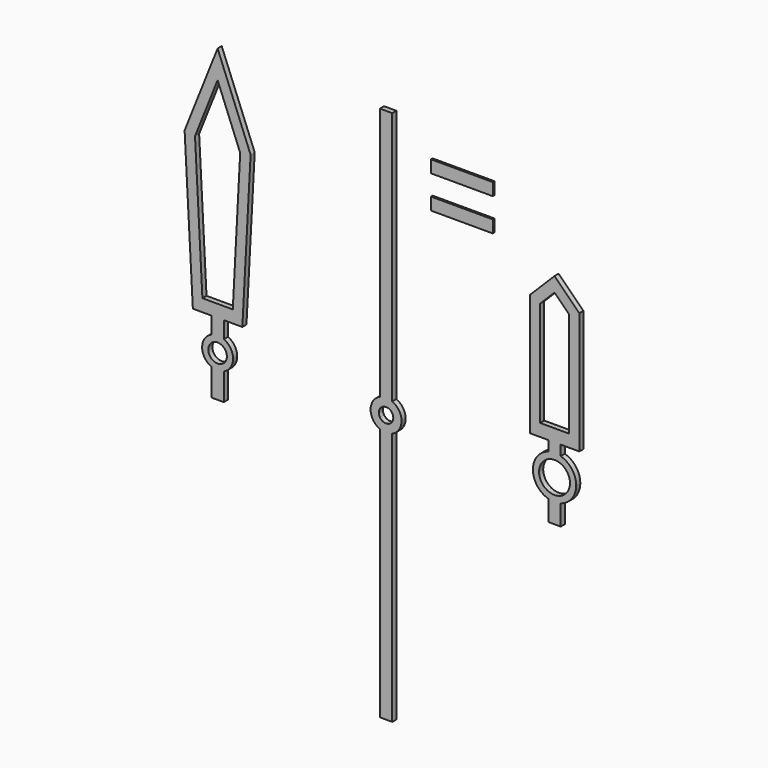
from build123d import *

# Parameters (mm, degrees)
F0_W     = 0.5
F0_H     = 0.6
F1_DEPTH = 0.25
F0_W_2   = 3
F2_DEPTH = 0.1


# Not quite as in the source:
# - a feature names something its author has since deleted; it is built from what else it names


with BuildPart() as f1:
    # F0 (on Front) → F1 (new body)
    with BuildSketch(Plane.XZ):
        with BuildLine():
            ThreePointArc((-20.5497518182, 1.0062305899), (-21.0916247302, 0.6274950199), (-21.2997518182, 0))
            Line((-21.2997518182, 0), (-20.9997518182, 0))
            ThreePointArc((-20.9997518182, 0), (-20.7800819041, 0.5303300859), (-20.2497518182, 0.75))
            Line((-20.2497518182, 0.75), (-20.2497518182, 1.05))
            ThreePointArc((-20.2497518182, 1.05), (-20.4013398794, 1.0390000287), (-20.5497518182, 1.0062305899))
        make_face()
        with BuildLine():
            Line((-20.9997518182, 0), (-21.2997518182, 0))
            ThreePointArc((-21.2997518182, 0), (-21.0916247302, -0.6274950199), (-20.5497518182, -1.0062305899))
            ThreePointArc((-20.5497518182, -1.0062305899), (-20.2497518182, -1.05), (-19.9497518182, -1.0062305899))
            ThreePointArc((-19.9497518182, -1.0062305899), (-19.4078789062, -0.6274950199), (-19.1997518182, 0))
            ThreePointArc((-19.1997518182, 0), (-19.4078789062, 0.6274950199), (-19.9497518182, 1.0062305899))
            ThreePointArc((-19.9497518182, 1.0062305899), (-20.0981637569, 1.0390000287), (-20.2497518182, 1.05))
            Line((-20.2497518182, 1.05), (-20.2497518182, 0.75))
            ThreePointArc((-20.2497518182, 0.75), (-19.7194217323, 0.5303300859), (-19.4997518182, 0))
            ThreePointArc((-19.4997518182, 0), (-20.2497518182, -0.75), (-20.9997518182, 0))
        make_face()
        with BuildLine():
            Line((-20.5497518182, 1.5), (-20.5497518182, 1.0062305899))
            ThreePointArc((-20.5497518182, 1.0062305899), (-20.4013398794, 1.0390000287), (-20.2497518182, 1.05))
            Line((-20.2497518182, 1.05), (-20.2497518182, 1.5))
            Line((-20.2497518182, 1.5), (-20.5497518182, 1.5))
        make_face()
        with BuildLine():
            ThreePointArc((-19.9497518182, -1.0062305899), (-20.2497518182, -1.05), (-20.5497518182, -1.0062305899))
            Line((-20.5497518182, -1.0062305899), (-20.5497518182, -2))
            Line((-20.5497518182, -2), (-19.9497518182, -2))
            Line((-19.9497518182, -2), (-19.9497518182, -1.0062305899))
        make_face()
        with BuildLine():
            Line((-20.2497518182, 1.5), (-20.2497518182, 1.05))
            ThreePointArc((-20.2497518182, 1.05), (-20.0981637569, 1.0390000287), (-19.9497518182, 1.0062305899))
            Line((-19.9497518182, 1.0062305899), (-19.9497518182, 1.5))
            Line((-19.9497518182, 1.5), (-20.2497518182, 1.5))
        make_face()
        Polygon((-20.9497518182, 1.5), (-20.5497518182, 1.5), (-20.2497518182, 1.5), (-20.2497518182, 2.1), (-20.9497518182, 2.1), align=None)
        Polygon((-20.2497518182, 2.1), (-20.2497518182, 1.5), (-19.9497518182, 1.5), (-19.5497518182, 1.5), (-19.5497518182, 2.1), align=None)
        with Locations((-21.1997518182, 1.8)):
            Rectangle(F0_W, F0_H)
        Polygon((-21.4497518182, 2.1), (-20.9497518182, 2.1), (-20.9497518182, 7.1928932188), (-20.2497518182, 7.8928932188), (-20.2497518182, 8.6), (-21.4497518182, 7.4), align=None)
        with Locations((-19.2997518182, 1.8)):
            Rectangle(F0_W, F0_H)
        Polygon((-20.2497518182, 8.6), (-20.2497518182, 7.8928932188), (-19.5497518182, 7.1928932188), (-19.5497518182, 2.1), (-19.0497518182, 2.1), (-19.0497518182, 7.4), align=None)
    extrude(amount=F1_DEPTH)


with BuildPart() as f1b:
    # F0 (on Front) → F1, piece 2 (new body)
    with BuildSketch(Plane.XZ):
        with BuildLine():
            ThreePointArc((-28.7187018186, 0.6873863542), (-29.0461968385, 0.4107919181), (-29.1687018186, 0))
            Line((-29.1687018186, 0), (-28.7687018186, 0))
            ThreePointArc((-28.7687018186, 0), (-28.7559702577, 0.0935414347), (-28.7187018186, 0.1802775638))
            Line((-28.7187018186, 0.1802775638), (-28.7187018186, 0.6873863542))
        make_face()
        with BuildLine():
            Line((-28.7687018186, 0), (-29.1687018186, 0))
            ThreePointArc((-29.1687018186, 0), (-29.0461968385, -0.4107919181), (-28.7187018186, -0.6873863542))
            Line((-28.7187018186, -0.6873863542), (-28.7187018186, -0.1802775638))
            ThreePointArc((-28.7187018186, -0.1802775638), (-28.7559702577, -0.0935414347), (-28.7687018186, 0))
        make_face()
        with BuildLine():
            Line((-28.7187018186, 12.9938064694), (-28.7187018186, 0.6873863542))
            ThreePointArc((-28.7187018186, 0.6873863542), (-28.5719340514, 0.7341797347), (-28.4187018186, 0.75))
            Line((-28.4187018186, 0.75), (-28.4187018186, 12.9938064694))
            Line((-28.4187018186, 12.9938064694), (-28.7187018186, 12.9938064694))
        make_face()
        with BuildLine():
            ThreePointArc((-28.4187018186, 0.75), (-28.5719340514, 0.7341797347), (-28.7187018186, 0.6873863542))
            Line((-28.7187018186, 0.6873863542), (-28.7187018186, 0.1802775638))
            ThreePointArc((-28.7187018186, 0.1802775638), (-28.5910428362, 0.3046285831), (-28.4187018186, 0.35))
            Line((-28.4187018186, 0.35), (-28.4187018186, 0.75))
        make_face()
        with BuildLine():
            Line((-28.7187018186, -0.1802775638), (-28.7187018186, -0.6873863542))
            ThreePointArc((-28.7187018186, -0.6873863542), (-28.5719340514, -0.7341797347), (-28.4187018186, -0.75))
            Line((-28.4187018186, -0.75), (-28.4187018186, -0.35))
            ThreePointArc((-28.4187018186, -0.35), (-28.5910428362, -0.3046285831), (-28.7187018186, -0.1802775638))
        make_face()
        with BuildLine():
            ThreePointArc((-28.4187018186, -0.75), (-28.5719340514, -0.7341797347), (-28.7187018186, -0.6873863542))
            Line((-28.7187018186, -0.6873863542), (-28.7187018186, -12.9938064694))
            Line((-28.7187018186, -12.9938064694), (-28.4187018186, -12.9938064694))
            Line((-28.4187018186, -12.9938064694), (-28.4187018186, -0.75))
        make_face()
        with BuildLine():
            Line((-28.4187018186, 12.9938064694), (-28.4187018186, 0.75))
            ThreePointArc((-28.4187018186, 0.75), (-28.2654695858, 0.7341797347), (-28.1187018186, 0.6873863542))
            Line((-28.1187018186, 0.6873863542), (-28.1187018186, 12.9938064694))
            Line((-28.1187018186, 12.9938064694), (-28.4187018186, 12.9938064694))
        make_face()
        with BuildLine():
            ThreePointArc((-28.1187018186, 0.6873863542), (-28.2654695858, 0.7341797347), (-28.4187018186, 0.75))
            Line((-28.4187018186, 0.75), (-28.4187018186, 0.35))
            ThreePointArc((-28.4187018186, 0.35), (-28.246360801, 0.3046285831), (-28.1187018186, 0.1802775638))
            Line((-28.1187018186, 0.1802775638), (-28.1187018186, 0.6873863542))
        make_face()
        with BuildLine():
            Line((-28.4187018186, -0.35), (-28.4187018186, -0.75))
            ThreePointArc((-28.4187018186, -0.75), (-28.2654695858, -0.7341797347), (-28.1187018186, -0.6873863542))
            Line((-28.1187018186, -0.6873863542), (-28.1187018186, -0.1802775638))
            ThreePointArc((-28.1187018186, -0.1802775638), (-28.246360801, -0.3046285831), (-28.4187018186, -0.35))
        make_face()
        with BuildLine():
            ThreePointArc((-28.1187018186, -0.6873863542), (-28.2654695858, -0.7341797347), (-28.4187018186, -0.75))
            Line((-28.4187018186, -0.75), (-28.4187018186, -12.9938064694))
            Line((-28.4187018186, -12.9938064694), (-28.1187018186, -12.9938064694))
            Line((-28.1187018186, -12.9938064694), (-28.1187018186, -0.6873863542))
        make_face()
        with BuildLine():
            ThreePointArc((-27.6687018186, 0), (-27.7912067987, 0.4107919181), (-28.1187018186, 0.6873863542))
            Line((-28.1187018186, 0.6873863542), (-28.1187018186, 0.1802775638))
            ThreePointArc((-28.1187018186, 0.1802775638), (-28.0814333795, 0.0935414347), (-28.0687018186, 0))
            Line((-28.0687018186, 0), (-27.6687018186, 0))
        make_face()
        with BuildLine():
            Line((-28.1187018186, -0.1802775638), (-28.1187018186, -0.6873863542))
            ThreePointArc((-28.1187018186, -0.6873863542), (-27.7912067987, -0.4107919181), (-27.6687018186, 0))
            Line((-27.6687018186, 0), (-28.0687018186, 0))
            ThreePointArc((-28.0687018186, 0), (-28.0814333795, -0.0935414347), (-28.1187018186, -0.1802775638))
        make_face()
    extrude(amount=F1_DEPTH)


with BuildPart() as f1c:
    # F0 (on Front) → F1, piece 3 (new body)
    with BuildSketch(Plane.XZ):
        Polygon((-34.987651819, 8.9829219505), (-36.587651819, 13), (-36.587651819, 11.6487521661), (-35.4928014695, 8.8999400996), (-35.850947132, 2.1), (-36.587651819, 2.1), (-36.587651819, 1.5), (-36.287651819, 1.5), (-35.387651819, 1.5), align=None)
        Polygon((-36.587651819, 11.6487521661), (-36.587651819, 13), (-38.187651819, 8.9829219505), (-37.787651819, 1.5), (-36.887651819, 1.5), (-36.587651819, 1.5), (-36.587651819, 2.1), (-37.3243565059, 2.1), (-37.6825021685, 8.8999400996), align=None)
        with BuildLine():
            Line((-36.287651819, 0.6873863542), (-36.287651819, 1.5))
            Line((-36.287651819, 1.5), (-36.587651819, 1.5))
            Line((-36.587651819, 1.5), (-36.587651819, 0.75))
            ThreePointArc((-36.587651819, 0.75), (-36.4344195862, 0.7341797347), (-36.287651819, 0.6873863542))
        make_face()
        with BuildLine():
            Line((-36.587651819, 0.75), (-36.587651819, 1.5))
            Line((-36.587651819, 1.5), (-36.887651819, 1.5))
            Line((-36.887651819, 1.5), (-36.887651819, 0.6873863542))
            ThreePointArc((-36.887651819, 0.6873863542), (-36.7408840518, 0.7341797347), (-36.587651819, 0.75))
        make_face()
        with BuildLine():
            ThreePointArc((-35.837651819, 0), (-35.9601567991, 0.4107919181), (-36.287651819, 0.6873863542))
            ThreePointArc((-36.287651819, 0.6873863542), (-36.4344195862, 0.7341797347), (-36.587651819, 0.75))
            Line((-36.587651819, 0.75), (-36.587651819, 0.45))
            ThreePointArc((-36.587651819, 0.45), (-36.2694537675, 0.3181980515), (-36.137651819, 0))
            Line((-36.137651819, 0), (-35.837651819, 0))
        make_face()
        with BuildLine():
            Line((-36.587651819, 0.45), (-36.587651819, 0.75))
            ThreePointArc((-36.587651819, 0.75), (-36.7408840518, 0.7341797347), (-36.887651819, 0.6873863542))
            ThreePointArc((-36.887651819, 0.6873863542), (-37.337651819, 0), (-36.887651819, -0.6873863542))
            ThreePointArc((-36.887651819, -0.6873863542), (-36.587651819, -0.75), (-36.287651819, -0.6873863542))
            ThreePointArc((-36.287651819, -0.6873863542), (-35.9601567991, -0.4107919181), (-35.837651819, 0))
            Line((-35.837651819, 0), (-36.137651819, 0))
            ThreePointArc((-36.137651819, 0), (-36.9058498705, -0.3181980515), (-36.587651819, 0.45))
        make_face()
        with BuildLine():
            ThreePointArc((-36.287651819, -0.6873863542), (-36.587651819, -0.75), (-36.887651819, -0.6873863542))
            Line((-36.887651819, -0.6873863542), (-36.887651819, -2))
            Line((-36.887651819, -2), (-36.287651819, -2))
            Line((-36.287651819, -2), (-36.287651819, -0.6873863542))
        make_face()
    extrude(amount=F1_DEPTH)


with BuildPart() as f1d:
    # F0 (on Front) → F1, piece 4 (new body)
    with BuildSketch(Plane.XZ):
        with Locations((-24.663922295, 11.3997036099)):
            Rectangle(F0_W_2, F0_H)
    extrude(amount=F1_DEPTH)


with BuildPart() as f1e:
    # F0 (on Front) → F1, piece 5 (new body)
    with BuildSketch(Plane.XZ):
        with Locations((-24.663922295, 9.8090009272)):
            Rectangle(F0_W_2, F0_H)
    extrude(amount=F1_DEPTH)


with BuildPart() as f2:
    # F2 (new): a face of the model
    f2_faces = [f1d.part.faces().sort_by_distance(p)[0] for p in [
        (-24.663922295, -0.25, 11.3997036099),
    ]]
    extrude(f2_faces, amount=F2_DEPTH)


with BuildPart() as f2b:
    # F2#2 (new): a face of the model
    f2_2_faces = [f1e.part.faces().sort_by_distance(p)[0] for p in [
        (-24.663922295, -0.25, 9.8090009272),
    ]]
    extrude(f2_2_faces, amount=F2_DEPTH)


solid = Compound([f1.part, f1b.part, f1c.part, f2.part, f2b.part])
